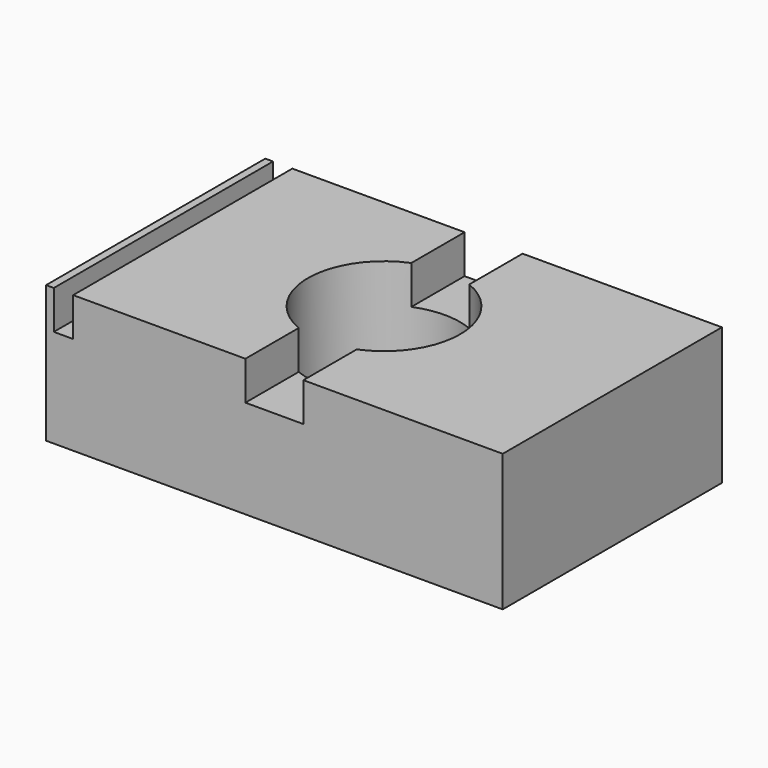
from build123d import *

# Parameters (mm, degrees)
F0_W     = 150
F0_H     = 90
F0_R     = 25
F1_DEPTH = 45
F2_W     = 6.35
F2_H     = 90
F3_DEPTH = 12.7


# Not quite as in the source:
# - a feature names something its author has since deleted; it is built from what else it names


with BuildPart() as f1:
    # F0 (on Top) → F1 (new body)
    with BuildSketch(Plane.XY):
        Rectangle(F0_W, F0_H)
        Circle(F0_R, mode=Mode.SUBTRACT)
    extrude(amount=F1_DEPTH)

    # F2 (on face) → F3 (cut)
    with BuildSketch(Plane.XY.offset(45)):
        with Locations((-69.285, 0)):
            Rectangle(F2_W, F2_H)
        with BuildLine():
            Line((-9.525, -23.1143759379), (-9.525, -45))
            Line((-9.525, -45), (9.525, -45))
            Line((9.525, -45), (9.525, -23.1143759379))
            ThreePointArc((9.525, -23.1143759379), (0, -25), (-9.525, -23.1143759379))
        make_face()
        with BuildLine():
            Line((9.525, 45), (-9.525, 45))
            Line((-9.525, 45), (-9.525, 23.1143759379))
            ThreePointArc((-9.525, 23.1143759379), (0, 25), (9.525, 23.1143759379))
            Line((9.525, 23.1143759379), (9.525, 45))
        make_face()
    extrude(amount=-F3_DEPTH, mode=Mode.SUBTRACT)


solid = f1.part
